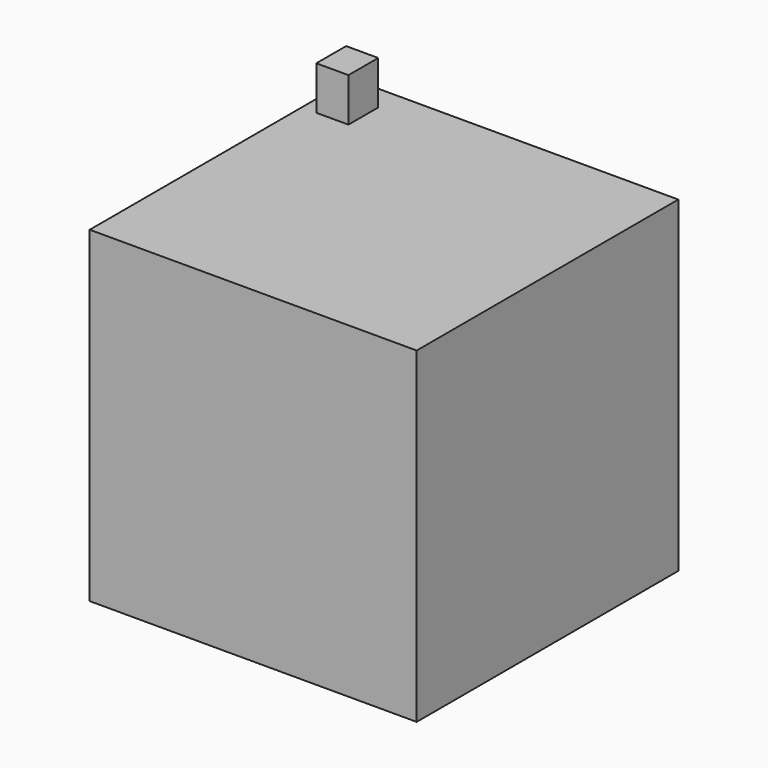
from build123d import *

# Parameters (mm, degrees)
F1_W     = 38.1
F1_H     = 38.1
F2_DEPTH = 19.05
F3_W     = 3.7443088368
F3_H     = 4.3355179951
F4_DEPTH = 5.08


# Not quite as in the source:
# - a variable given as a bare number and used for a length is read in inches; the dataset says mm whatever the document's units were


with BuildPart() as f2:
    # F1 (on Top) → F2 (new body, symmetric)
    with BuildSketch(Plane.XY):
        Rectangle(F1_W, F1_H)
    extrude(amount=F2_DEPTH, both=True)

    # F3 (on face) → F4 (join)
    with BuildSketch(Plane.XY.offset(19.05)):
        with Locations((-15.4699138366, 13.9918965288)):
            Rectangle(F3_W, F3_H)
    extrude(amount=F4_DEPTH)


solid = f2.part
